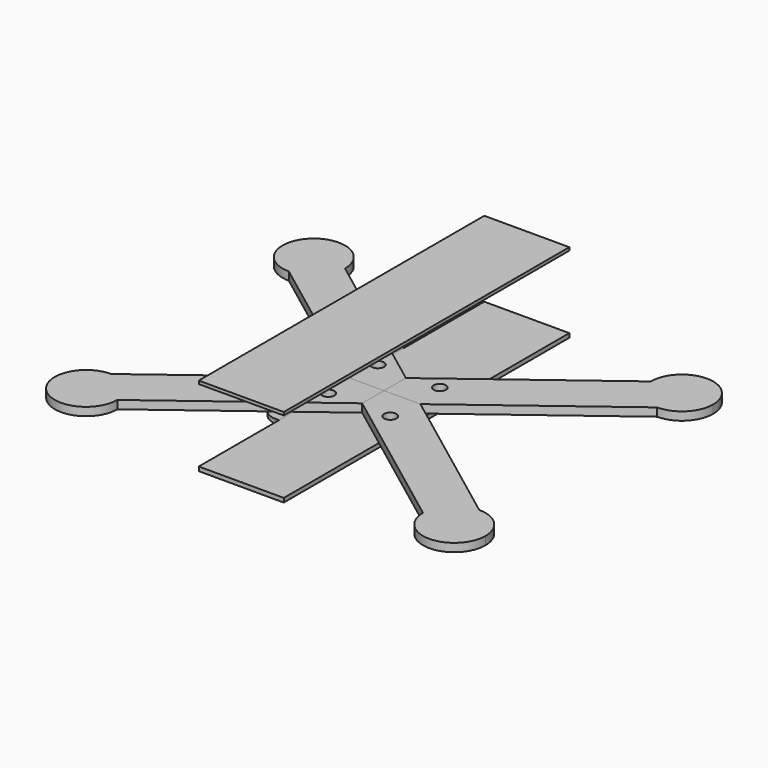
from build123d import *

# Parameters (mm, degrees)
F0_W           = 41.15
F0_H           = 172.72
F1_DEPTH       = 2
F3_START       = 2
F3_DEPTH       = 4
F4_START       = 2
F4_DEPTH       = 4
F5_START       = 2
F5_DEPTH       = 4
F6_START       = 2
F6_DEPTH       = 4
F8_START       = 37.108
F7_W           = 41.15
F7_H           = 172.72
F8_DEPTH       = 1.5
F9_R           = 3
F10_DEPTH      = 2
F10_DEPTH_BACK = 8
F11_W          = 41.15
F11_H          = 75.6703085505
F12_DEPTH      = 2


# Not quite as in the source:
# - a feature names something its author has since deleted; it is built from what else it names


with BuildPart() as f1:
    # F0 (on Top) → F1 (new body)
    with BuildSketch(Plane.XY):
        Rectangle(F0_W, F0_H)
    extrude(amount=F1_DEPTH)


with BuildPart() as f3:
    # F2 (on Top) → F3 (new body)
    with BuildSketch(Plane.XY.offset(F3_START)):
        Polygon((0.1391619444, -0.1772679389), (-17.4635283139, -0.1772679389), (0.1391619444, -13.4175834731), align=None)
        with BuildLine():
            Line((0.1391619444, -13.4175834731), (-17.4635283139, -0.1772679389))
            Line((-17.4635283139, -0.1772679389), (-88.9506042004, -53.9481079335))
            ThreePointArc((-88.9506042004, -53.9481079335), (-78.2640994163, -58.3746031494), (-73.8376042004, -69.0611079335))
            Line((-73.8376042004, -69.0611079335), (0.1391619444, -13.4175834731))
        make_face()
        with BuildLine():
            ThreePointArc((-73.8376042004, -69.0611079335), (-78.2640994163, -58.3746031494), (-88.9506042004, -53.9481079335))
            ThreePointArc((-88.9506042004, -53.9481079335), (-99.6371089844, -79.7476127176), (-73.8376042004, -69.0611079335))
        make_face()
    extrude(amount=F3_DEPTH)


with BuildPart() as f4:
    # F2 (on Top) → F4 (new body)
    with BuildSketch(Plane.XY.offset(F4_START)):
        with BuildLine():
            ThreePointArc((104.3419280891, -69.0611079335), (99.9154328732, -58.3746031494), (89.2289280891, -53.9481079335))
            ThreePointArc((89.2289280891, -53.9481079335), (78.5424233051, -58.3746031494), (74.1159280891, -69.0611079335))
            ThreePointArc((74.1159280891, -69.0611079335), (89.2289280891, -84.1741079335), (104.3419280891, -69.0611079335))
        make_face()
        with BuildLine():
            Line((89.2289280891, -53.9481079335), (17.7418522027, -0.1772679389))
            Line((17.7418522027, -0.1772679389), (0.1391619444, -13.4175834731))
            Line((0.1391619444, -13.4175834731), (74.1159280891, -69.0611079335))
            ThreePointArc((74.1159280891, -69.0611079335), (78.5424233051, -58.3746031494), (89.2289280891, -53.9481079335))
        make_face()
        Polygon((0.1391619444, -13.4175834731), (17.7418522027, -0.1772679389), (0.1391619444, -0.1772679389), align=None)
    extrude(amount=F4_DEPTH)


with BuildPart() as f5:
    # F2 (on Top) → F5 (new body)
    with BuildSketch(Plane.XY.offset(F5_START)):
        with BuildLine():
            ThreePointArc((104.3419280891, 68.7065720558), (89.2289280891, 83.8195720558), (74.1159280891, 68.7065720558))
            ThreePointArc((74.1159280891, 68.7065720558), (78.5424233051, 58.0200672717), (89.2289280891, 53.5935720558))
            ThreePointArc((89.2289280891, 53.5935720558), (99.9154328732, 58.0200672717), (104.3419280891, 68.7065720558))
        make_face()
        with BuildLine():
            Line((74.1159280891, 68.7065720558), (0.1391619444, 13.0630475954))
            Line((0.1391619444, 13.0630475954), (17.7418522027, -0.1772679389))
            Line((17.7418522027, -0.1772679389), (89.2289280891, 53.5935720558))
            ThreePointArc((89.2289280891, 53.5935720558), (78.5424233051, 58.0200672717), (74.1159280891, 68.7065720558))
        make_face()
        Polygon((17.7418522027, -0.1772679389), (0.1391619444, 13.0630475954), (0.1391619444, -0.1772679389), align=None)
    extrude(amount=F5_DEPTH)


with BuildPart() as f6:
    # F2 (on Top) → F6 (new body)
    with BuildSketch(Plane.XY.offset(F6_START)):
        with BuildLine():
            ThreePointArc((-88.9506042004, 53.5935720558), (-78.2640994163, 58.0200672717), (-73.8376042004, 68.7065720558))
            ThreePointArc((-73.8376042004, 68.7065720558), (-99.6371089844, 79.3930768399), (-88.9506042004, 53.5935720558))
        make_face()
        with BuildLine():
            Line((0.1391619444, 13.0630475954), (-73.8376042004, 68.7065720558))
            ThreePointArc((-73.8376042004, 68.7065720558), (-78.2640994163, 58.0200672717), (-88.9506042004, 53.5935720558))
            Line((-88.9506042004, 53.5935720558), (-17.4635283139, -0.1772679389))
            Line((-17.4635283139, -0.1772679389), (0.1391619444, 13.0630475954))
        make_face()
        Polygon((0.1391619444, -0.1772679389), (0.1391619444, 13.0630475954), (-17.4635283139, -0.1772679389), align=None)
    extrude(amount=F6_DEPTH)


with BuildPart() as f8:
    # F7 (on Top) → F8 (new body)
    with BuildSketch(Plane.XY.offset(F8_START)):
        Rectangle(F7_W, F7_H)
    extrude(amount=F8_DEPTH)


with BuildPart() as f10_tool:
    # F9 (on face) → F10 (new body, two sides)
    with BuildSketch(Plane.XY) as f10_sk:
        with Locations((15, 15)):
            Circle(F9_R)
        with Locations((15, -15)):
            Circle(F9_R)
        with Locations((-15, -15)):
            Circle(F9_R)
        with Locations((-15, 15)):
            Circle(F9_R)
    extrude(amount=-F10_DEPTH)
    extrude(f10_sk.sketch, amount=F10_DEPTH_BACK)


with BuildPart() as f1_1:
    add(f1.part)

    # F10: cut by f10_tool
    add(f10_tool.part, mode=Mode.SUBTRACT)


with BuildPart() as f3_1:
    add(f3.part)

    # F10: cut by f10_tool
    add(f10_tool.part, mode=Mode.SUBTRACT)


with BuildPart() as f4_1:
    add(f4.part)

    # F10: cut by f10_tool
    add(f10_tool.part, mode=Mode.SUBTRACT)


with BuildPart() as f5_1:
    add(f5.part)

    # F10: cut by f10_tool
    add(f10_tool.part, mode=Mode.SUBTRACT)


with BuildPart() as f6_1:
    add(f6.part)

    # F10: cut by f10_tool
    add(f10_tool.part, mode=Mode.SUBTRACT)


with BuildPart() as f12:
    # F11 (on face) → F12 (new body)
    with BuildSketch(Plane.XY):
        with BuildLine():
            Line((-20.575, 37.8859647318), (-22.3068072487, 37.8859647318))
            ThreePointArc((-22.3068072487, 37.8859647318), (-27.9636614982, 35.5428189813), (-30.3068072487, 29.8859647318))
            Line((-30.3068072487, 29.8859647318), (-30.3068072487, 7.7289344695))
            Line((-30.3068072487, 7.7289344695), (-28.1127241634, 6.173899075))
            ThreePointArc((-28.1127241634, 6.173899075), (-25.1716069065, 0.8588809734), (-27.4934151644, -4.7543885332))
            Line((-27.4934151644, -4.7543885332), (-30.3068072487, -7.2710655305))
            Line((-30.3068072487, -7.2710655305), (-30.3068072487, -29.7843438187))
            ThreePointArc((-30.3068072487, -29.7843438187), (-27.9636614982, -35.4411980681), (-22.3068072487, -37.7843438187))
            Line((-22.3068072487, -37.7843438187), (-20.575, -37.7843438187))
            Line((-20.575, -37.7843438187), (-20.575, 37.8859647318))
        make_face()
        with Locations((0, 0.0508104566)):
            Rectangle(F11_W, F11_H)
    extrude(amount=F12_DEPTH)


with BuildPart() as f12b:
    # F0 (on Top) → F12, piece 2 (new body)
    with BuildSketch(Plane.XY):
        Rectangle(F0_W, F0_H)
    extrude(amount=F12_DEPTH)


solid = Compound([f8.part, f1_1.part, f3_1.part, f4_1.part, f5_1.part, f6_1.part, f12.part, f12b.part])
